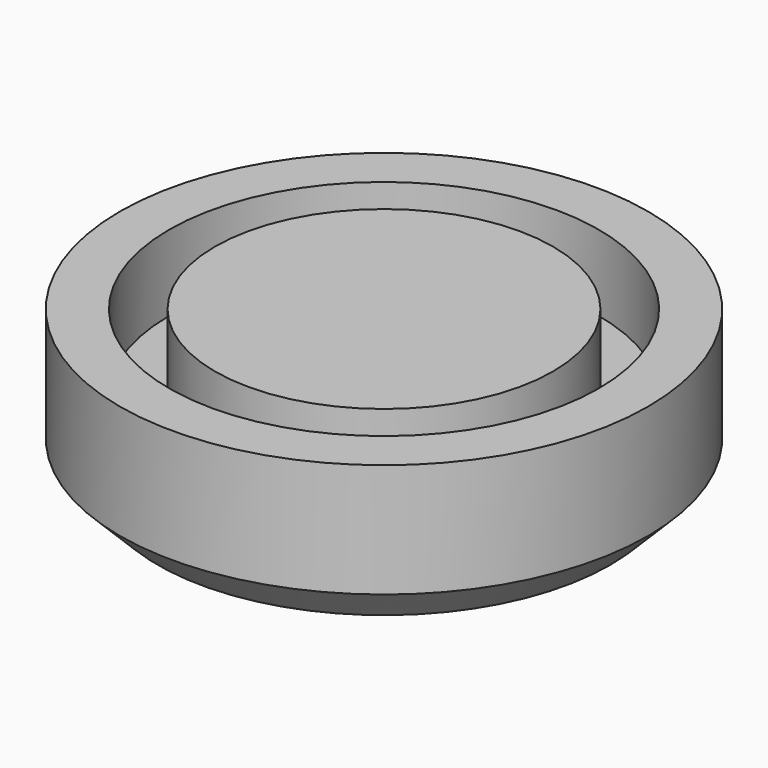
from build123d import *

# Parameters (mm, degrees)
F0_R     = 707.076711983
F0_R_2   = 575.1975047279
F0_R_3   = 452.5428910843
F1_DEPTH = 203.2
F2_DEPTH = 203.2
F3_SIZE  = 101.6


# Not quite as in the source:
# - a feature names something its author has since deleted; it is built from what else it names


with BuildPart() as f1:
    # F0 (on Top) → F1 (new body)
    with BuildSketch(Plane.XY):
        Circle(F0_R)
        Circle(F0_R_2, mode=Mode.SUBTRACT)
        Circle(F0_R_2)
        Circle(F0_R_3, mode=Mode.SUBTRACT)
        Circle(F0_R_3)
    extrude(amount=-F1_DEPTH)

    # F0 (on Top) → F2 (join)
    with BuildSketch(Plane.XY):
        Circle(F0_R)
        Circle(F0_R_2, mode=Mode.SUBTRACT)
        Circle(F0_R_3)
    extrude(amount=F2_DEPTH)

    # F3
    f3_edges = [f1.edges().sort_by_distance(p)[0] for p in [
        (-707.076712, 0, -203.2),
    ]]
    chamfer(f3_edges, length=F3_SIZE)


solid = f1.part
